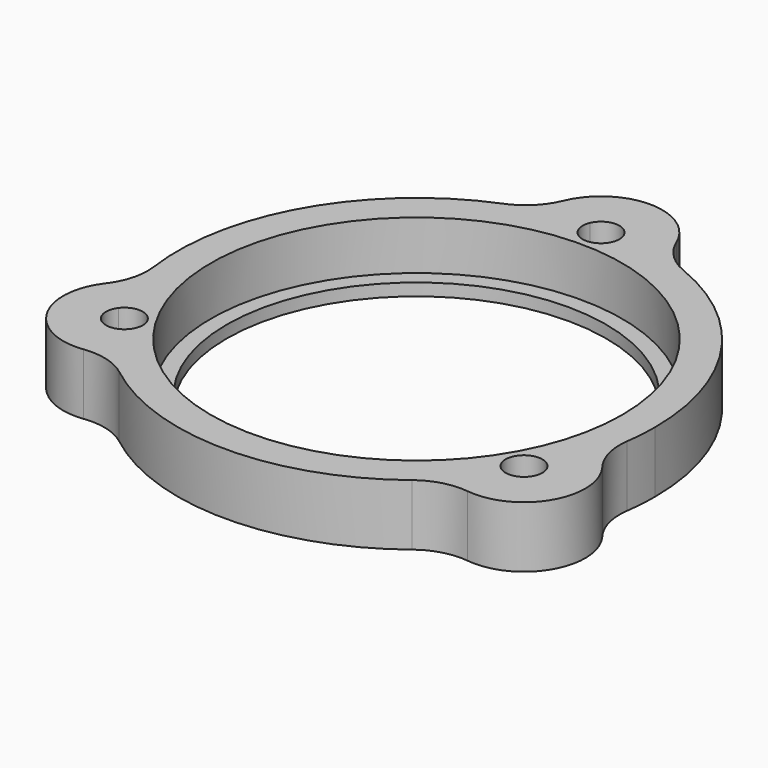
from build123d import *

# Parameters (mm, degrees)
F0_R     = 21.336
F0_R_2   = 19.685
F1_DEPTH = 1.27
F2_DEPTH = 6.35
F3_R     = 6.35


with BuildPart() as f1:
    # F0 (on Top) → F1 (new body)
    with BuildSketch(Plane.XY):
        Circle(F0_R)
        Circle(F0_R_2, mode=Mode.SUBTRACT)
    extrude(amount=F1_DEPTH)

    # F0 (on Top) → F2 (join)
    with BuildSketch(Plane.XY):
        with BuildLine():
            ThreePointArc((23.9050999455, -6.4692674698), (24.5490837421, -3.2630832697), (24.765, 0))
            ThreePointArc((24.765, 0), (19.6285885254, 15.1004548773), (6.35, 23.9370575677))
            ThreePointArc((6.35, 23.9370575677), (4.0651088886, 24.4290833787), (1.7440091422, 24.703515076))
            ThreePointArc((1.7440091422, 24.703515076), (1.8643178935, 24.3286489263), (1.905, 23.9370575677))
            ThreePointArc((1.905, 23.9370575677), (-0.3915913586, 22.0727396742), (-1.7440091422, 24.703515076))
            ThreePointArc((-1.7440091422, 24.703515076), (-4.0651088886, 24.4290833787), (-6.35, 23.9370575677))
            ThreePointArc((-6.35, 23.9370575677), (-21.4471191247, 12.3825), (-23.9050999455, -6.4692674698))
            ThreePointArc((-23.9050999455, -6.4692674698), (-23.1887612414, -8.6940541227), (-22.2658761897, -10.8414013165))
            ThreePointArc((-22.2658761897, -10.8414013165), (-20.1370690632, -10.1581864481), (-18.8250999455, -11.9685287839))
            ThreePointArc((-18.8250999455, -11.9685287839), (-19.3113489683, -13.239815795), (-20.5218670475, -13.8621137596))
            ThreePointArc((-20.5218670475, -13.8621137596), (-19.1236523528, -15.735029256), (-17.5550999455, -17.4677900979))
            ThreePointArc((-17.5550999455, -17.4677900979), (0, -24.765), (17.5550999455, -17.4677900979))
            ThreePointArc((17.5550999455, -17.4677900979), (19.1236523528, -15.735029256), (20.5218670475, -13.8621137596))
            ThreePointArc((20.5218670475, -13.8621137596), (19.0803215513, -11.0160287839), (22.2658761897, -10.8414013165))
            ThreePointArc((22.2658761897, -10.8414013165), (23.1887612414, -8.6940541227), (23.9050999455, -6.4692674698))
        make_face()
        Circle(F0_R, mode=Mode.SUBTRACT)
        with BuildLine():
            ThreePointArc((1.7440091422, 24.703515076), (4.0651088886, 24.4290833787), (6.35, 23.9370575677))
            ThreePointArc((6.35, 23.9370575677), (0, 30.2870575677), (-6.35, 23.9370575677))
            ThreePointArc((-6.35, 23.9370575677), (-4.0651088886, 24.4290833787), (-1.7440091422, 24.703515076))
            ThreePointArc((-1.7440091422, 24.703515076), (0, 25.8420575677), (1.7440091422, 24.703515076))
        make_face()
        with BuildLine():
            ThreePointArc((17.5550999455, -17.4677900979), (26.2293612595, -15.1435287839), (23.9050999455, -6.4692674698))
            ThreePointArc((23.9050999455, -6.4692674698), (23.1887612414, -8.6940541227), (22.2658761897, -10.8414013165))
            ThreePointArc((22.2658761897, -10.8414013165), (22.5404422812, -11.3754979015), (22.6350999455, -11.9685287839))
            ThreePointArc((22.6350999455, -11.9685287839), (22.0013869566, -13.3872797611), (20.5218670475, -13.8621137596))
            ThreePointArc((20.5218670475, -13.8621137596), (19.1236523528, -15.735029256), (17.5550999455, -17.4677900979))
        make_face()
        with BuildLine():
            ThreePointArc((-22.2658761897, -10.8414013165), (-23.1887612414, -8.6940541227), (-23.9050999455, -6.4692674698))
            ThreePointArc((-23.9050999455, -6.4692674698), (-26.2293612595, -15.1435287839), (-17.5550999455, -17.4677900979))
            ThreePointArc((-17.5550999455, -17.4677900979), (-19.1236523528, -15.735029256), (-20.5218670475, -13.8621137596))
            ThreePointArc((-20.5218670475, -13.8621137596), (-22.3798783397, -12.9210287839), (-22.2658761897, -10.8414013165))
        make_face()
    extrude(amount=F2_DEPTH)

    # F3
    f3_edges = [f1.edges().sort_by_distance(p)[0] for p in [
        (6.35, 23.937058, 3.175),
        (-23.9051, -6.469267, 3.175),
        (17.5551, -17.46779, 3.175),
        (23.9051, -6.469267, 3.175),
        (-6.35, 23.937058, 3.175),
        (-17.5551, -17.46779, 3.175),
    ]]
    fillet(f3_edges, radius=F3_R)


solid = f1.part
